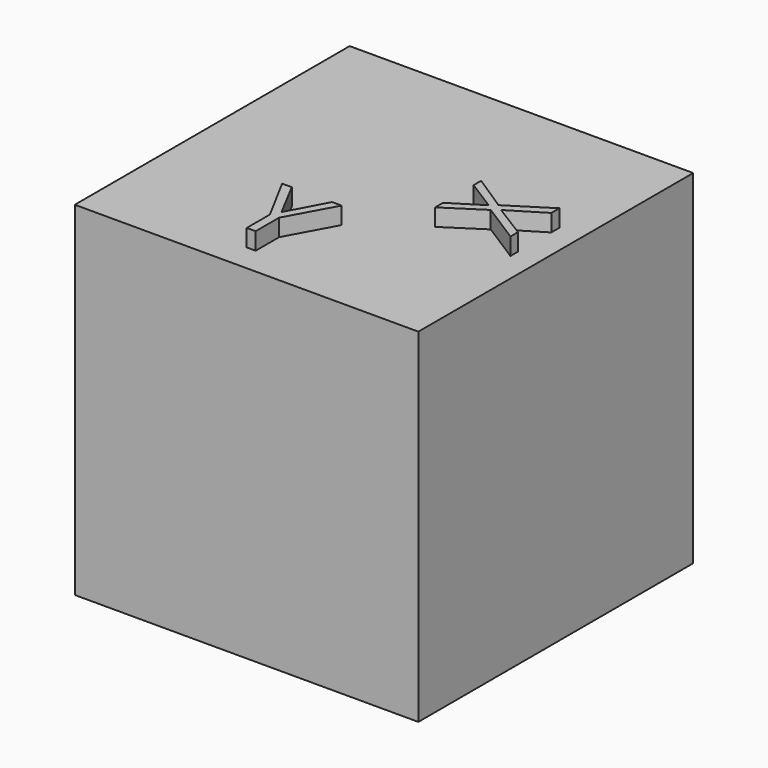
from build123d import *

# Parameters (mm, degrees)
F0_W           = 10
F0_H           = 10
F1_DEPTH       = 10
F2_TEXT_SIZE   = 3.0890126911
F2_TEXT_SIZE_2 = 3.1283350836
F3_DEPTH       = 0.5


# Not quite as in the source:
# - Text() gives the source's letters only with a copy of the font that has no kerning and outlines rounded to 1/6400 em; it was checked with that copy


with BuildPart() as f1:
    # F0 (on Top) → F1 (new body)
    with BuildSketch(Plane.XY):
        with Locations((3.904967336, -1.281589649)):
            Rectangle(F0_W, F0_H)
    extrude(amount=F1_DEPTH)

    # F2 (on face) → F3 (join)
    with BuildSketch(Plane.XY.offset(10)):
        with Locations((2.5354193058, -5.4815905169)):
            Text('Y', F2_TEXT_SIZE, font='Open Sans', text_align=(TextAlign.LEFT, TextAlign.BOTTOM))
        with Locations(Location((8.2140201121, -2.0798591431), (0, 0, 90))):
            Text('X', F2_TEXT_SIZE_2, font='Open Sans', text_align=(TextAlign.LEFT, TextAlign.BOTTOM))
    extrude(amount=F3_DEPTH)


solid = f1.part
